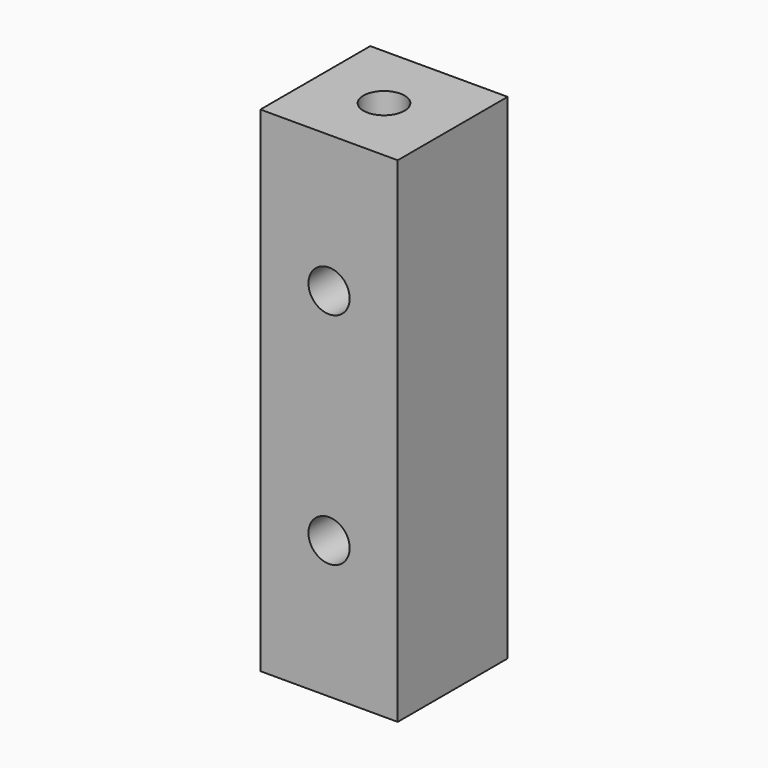
from build123d import *

# Parameters (mm, degrees)
F0_W     = 10
F0_H     = 10
F1_DEPTH = 18
F2_R     = 1.5
F3_DEPTH = 7.5
F4_R     = 1.5
F5_DEPTH = 12.5


# Not quite as in the source:
# - a pattern or mirror of a feature is missing from the dataset's text; its kind, count and spacing are read off the source's solid


with BuildPart() as f1:
    # F0 (on Top) → F1 (new body, symmetric)
    with BuildSketch(Plane.XY):
        Rectangle(F0_W, F0_H)
    extrude(amount=F1_DEPTH, both=True)

    # F2 (on face) → F3 (cut)
    with BuildSketch(Plane.XY.offset(18)):
        Circle(F2_R)
    f3 = extrude(amount=-F3_DEPTH, mode=Mode.SUBTRACT)

    # F3_copies: F3 across plane
    add(f3.mirror(Plane(origin=(0, 0, 0), x_dir=(-1, 0, 0), z_dir=(0, 0, -1))), mode=Mode.SUBTRACT)

    # F4 (on Front) → F5 (cut, symmetric)
    with BuildSketch(Plane.XZ):
        with Locations((0, 8)):
            Circle(F4_R)
    f5 = extrude(amount=F5_DEPTH, both=True, mode=Mode.SUBTRACT)

    # F5_copies: F5 across plane
    add(f5.mirror(Plane(origin=(0, 0, 0), x_dir=(-1, 0, 0), z_dir=(0, 0, -1))), mode=Mode.SUBTRACT)


solid = f1.part
